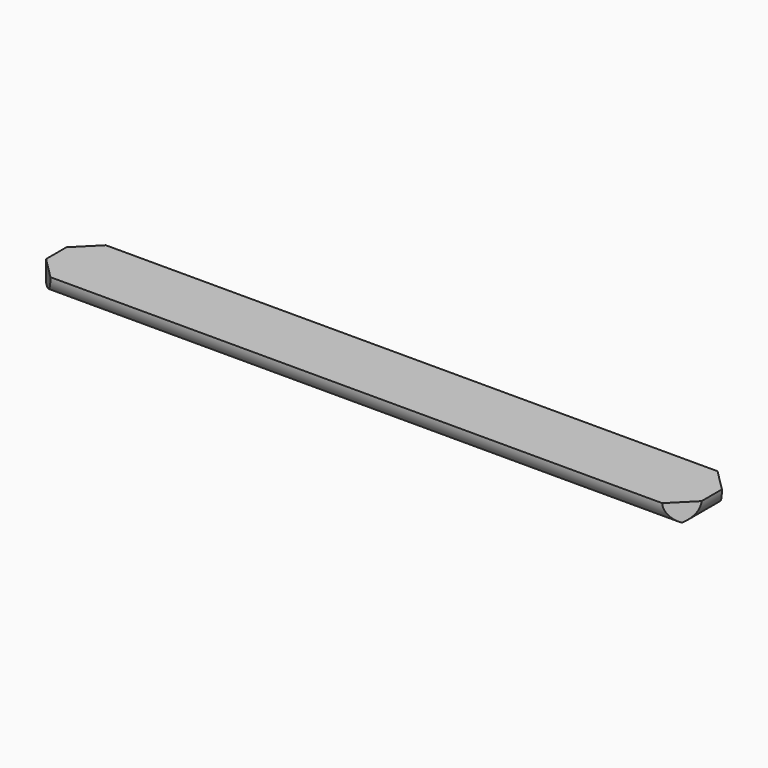
from build123d import *

# Parameters (mm, degrees)
F0_W        = 149.9416083097
F0_H        = 15.8279500902
F1_DEPTH    = 4.826
F2_SIZE     = 5
F3_T1_DEPTH = 164.9264657238
F4_T1_DEPTH = 164.9264657238
F5_T1_DEPTH = 30.8128075042


# Not quite as in the source:
# - a fillet or chamfer that OpenCascade refuses, or shapes differently, is made with other operations: its cross-section is extruded or revolved along the edge and cut away or added


with BuildPart() as f1:
    # F0 (on Top) → F1 (new body)
    with BuildSketch(Plane.XY):
        with Locations((-74.9708041549, 7.9139750451)):
            Rectangle(F0_W, F0_H)
    extrude(amount=F1_DEPTH)

    # F2
    f2_edges = [f1.edges().sort_by_distance(p)[0] for p in [
        (-149.941608, 15.82795, 2.413),
        (-149.941608, 0, 2.413),
        (0, 15.82795, 2.413),
        (0, 0, 2.413),
    ]]
    chamfer(f2_edges, length=F2_SIZE)

    # F3: fillet of radius 5 on 1 edges, made by hand

    # F3_s2 → F3_t1 (cut)
    with BuildSketch(Plane.YZ.offset(-157.4340370168)):
        with BuildLine():
            ThreePointArc((0, 4.826), (1.5235005962, 1.4034738983), (4.9969714828, 0))
            Line((4.9969714828, 0), (0, 0))
            Line((0, 0), (0, 4.826))
        make_face()
    extrude(amount=F3_T1_DEPTH, mode=Mode.SUBTRACT)

    # F4: fillet of radius 5 on 1 edges, made by hand

    # F4_s2 → F4_t1 (cut)
    with BuildSketch(Plane.YZ.offset(-157.4340370168)):
        with BuildLine():
            ThreePointArc((15.8279500902, 4.826), (14.304449494, 1.4034738983), (10.8309786074, 0))
            Line((10.8309786074, 0), (15.8279500902, 0))
            Line((15.8279500902, 0), (15.8279500902, 4.826))
        make_face()
    extrude(amount=F4_T1_DEPTH, mode=Mode.SUBTRACT)

    # F5: fillet of radius 5 on 1 edges, made by hand

    # F5_s2 → F5_t1 (cut)
    with BuildSketch(Plane.XZ.offset(-23.3203787972)):
        with BuildLine():
            ThreePointArc((0, 4.826), (-1.5235005962, 1.4034738983), (-4.9969714828, 0))
            Line((-4.9969714828, 0), (0, 0))
            Line((0, 0), (0, 4.826))
        make_face()
    extrude(amount=F5_T1_DEPTH, mode=Mode.SUBTRACT)


solid = f1.part
